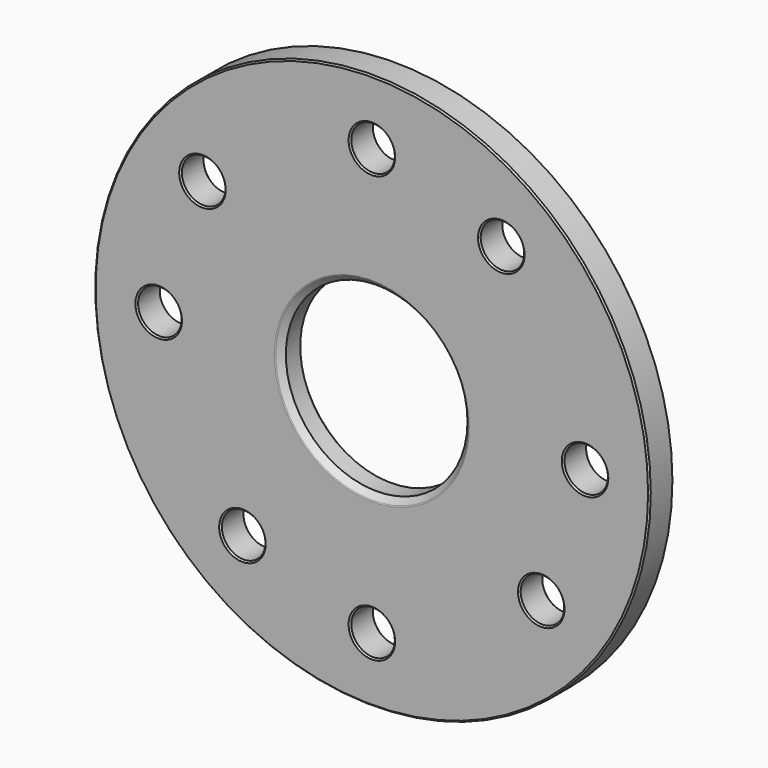
from build123d import *

# Parameters (mm, degrees)
F0_R     = 92.5
F0_R_2   = 7.25
F0_R_3   = 30.25
F1_DEPTH = 10
F2_SIZE2 = 2
F2_SIZE  = 2
F3_SIZE2 = 2
F3_SIZE  = 2


# Not quite as in the source:
# - a fillet or chamfer that OpenCascade refuses, or shapes differently, is made with other operations: its cross-section is extruded or revolved along the edge and cut away or added


with BuildPart() as f1:
    # F0 (on Front) → F1 (new body)
    with BuildSketch(Plane.XZ):
        Circle(F0_R)
        with BuildLine():
            ThreePointArc((-35.8509998507, -56.4207746479), (-35.9472026921, -57.5979263852), (-36.2332581163, -58.7438380282))
            ThreePointArc((-36.2332581163, -58.7438380282), (-50.2547970094, -55.2436229106), (-35.8509998507, -56.4207746479))
        make_face(mode=Mode.SUBTRACT)
        with BuildLine():
            ThreePointArc((-6.8677417345, -68.6769366197), (1.1771517373, -63.8462028413), (7.25, -71))
            ThreePointArc((7.25, -71), (-1.1771517373, -78.1537971587), (-6.8677417345, -68.6769366197))
        make_face(mode=Mode.SUBTRACT)
        with Locations((56.4207746479, -43.1009998507)):
            Circle(F0_R_2, mode=Mode.SUBTRACT)
        with Locations((-71, 0)):
            Circle(F0_R_2, mode=Mode.SUBTRACT)
        with Locations((-56.4207746479, 43.1009998507)):
            Circle(F0_R_2, mode=Mode.SUBTRACT)
        Circle(F0_R_3, mode=Mode.SUBTRACT)
        with Locations((71, 0)):
            Circle(F0_R_2, mode=Mode.SUBTRACT)
        with Locations((43.1009998507, 56.4207746479)):
            Circle(F0_R_2, mode=Mode.SUBTRACT)
        with Locations((0, 71)):
            Circle(F0_R_2, mode=Mode.SUBTRACT)
    extrude(amount=-F1_DEPTH)

    # F2
    f2_edges = [f1.edges().sort_by_distance(p)[0] for p in [
        (-30.25, 0, 0),
    ]]
    chamfer(f2_edges, length=F2_SIZE, length2=F2_SIZE2)

    # F3
    f3_edges = [f1.edges().sort_by_distance(p)[0] for p in [
        (-30.25, 10, 0),
    ]]
    chamfer(f3_edges, length=F3_SIZE, length2=F3_SIZE2)

    # F4: chamfer of 0.5 on 10 edges, made by hand

    # F4_s1 → F4_t2 (revolve, cut)
    with BuildSketch(Plane.XY):
        Polygon((32.1035533906, 9.8535533906), (32.4571067812, 10), (32.25, 10), align=None)
    revolve(axis=Axis((0, 10, 0), (0, -1, 0)), mode=Mode.SUBTRACT)

    # F4_s3 → F4_t4 (revolve, cut)
    with BuildSketch(Plane.XY):
        Polygon((92, 10), (92.5, 9.5), (92.5, 10), align=None)
    revolve(axis=Axis((0, 10, 0), (0, -1, 0)), mode=Mode.SUBTRACT)

    # F4_s5 → F4_t6 (revolve, cut)
    with BuildSketch(Plane.XY.offset(-56.4207746479)):
        Polygon((-35.3509998507, 10), (-35.8509998507, 9.5), (-35.8509998507, 10), align=None)
    revolve(axis=Axis((-43.1009998507, 10, -56.4207746479), (0, 1, 0)), mode=Mode.SUBTRACT)

    # F4_s7 → F4_t8 (revolve, cut)
    with BuildSketch(Plane(origin=(-21.5504999254, 0, -63.7103873239), x_dir=(0, 1, 0), z_dir=(-0.3204225352, 0, -0.947274722))):
        Polygon((10, 15), (9.5, 15.5), (10, 15.5), align=None)
    revolve(axis=Axis((0, 10, -71), (0, 1, 0)), mode=Mode.SUBTRACT)

    # F4_s9 → F4_t10 (revolve, cut)
    with BuildSketch(Plane.XY.offset(-43.1009998507)):
        Polygon((64.1707746479, 10), (63.6707746479, 9.5), (63.6707746479, 10), align=None)
    revolve(axis=Axis((56.4207746479, 10, -43.1009998507), (0, -1, 0)), mode=Mode.SUBTRACT)

    # F4_s11 → F4_t12 (revolve, cut)
    with BuildSketch(Plane.XY):
        Polygon((-63.25, 10), (-63.75, 9.5), (-63.75, 10), align=None)
    revolve(axis=Axis((-71, 10, 0), (0, -1, 0)), mode=Mode.SUBTRACT)

    # F4_s13 → F4_t14 (revolve, cut)
    with BuildSketch(Plane.XY.offset(43.1009998507)):
        Polygon((-48.6707746479, 10), (-49.1707746479, 9.5), (-49.1707746479, 10), align=None)
    revolve(axis=Axis((-56.4207746479, 10, 43.1009998507), (0, -1, 0)), mode=Mode.SUBTRACT)

    # F4_s15 → F4_t16 (revolve, cut)
    with BuildSketch(Plane.XY):
        Polygon((78.75, 10), (78.25, 9.5), (78.25, 10), align=None)
    revolve(axis=Axis((71, 10, 0), (0, -1, 0)), mode=Mode.SUBTRACT)

    # F4_s17 → F4_t18 (revolve, cut)
    with BuildSketch(Plane.XY.offset(56.4207746479)):
        Polygon((50.8509998507, 10), (50.3509998507, 9.5), (50.3509998507, 10), align=None)
    revolve(axis=Axis((43.1009998507, 10, 56.4207746479), (0, -1, 0)), mode=Mode.SUBTRACT)

    # F4_s19 → F4_t20 (revolve, cut)
    with BuildSketch(Plane.XY.offset(71)):
        Polygon((7.75, 10), (7.25, 9.5), (7.25, 10), align=None)
    revolve(axis=Axis((0, 10, 71), (0, -1, 0)), mode=Mode.SUBTRACT)

    # F5: chamfer of 0.5 on 10 edges, made by hand

    # F5_s1 → F5_t2 (revolve, cut)
    with BuildSketch(Plane.XY):
        Polygon((32.1035533906, 0.1464466094), (32.4571067812, 0), (32.25, 0), align=None)
    revolve(axis=Axis((0, 0, 0), (0, -1, 0)), mode=Mode.SUBTRACT)

    # F5_s3 → F5_t4 (revolve, cut)
    with BuildSketch(Plane.XY):
        Polygon((92, 0), (92.5, 0.5), (92.5, 0), align=None)
    revolve(axis=Axis((0, 0, 0), (0, -1, 0)), mode=Mode.SUBTRACT)

    # F5_s5 → F5_t6 (revolve, cut)
    with BuildSketch(Plane.XY.offset(-56.4207746479)):
        Polygon((-35.3509998507, 0), (-35.8509998507, 0.5), (-35.8509998507, 0), align=None)
    revolve(axis=Axis((-43.1009998507, 0, -56.4207746479), (0, -1, 0)), mode=Mode.SUBTRACT)

    # F5_s7 → F5_t8 (revolve, cut)
    with BuildSketch(Plane(origin=(-21.5504999254, 0, -63.7103873239), x_dir=(0, 1, 0), z_dir=(0.3204225352, 0, 0.947274722))):
        Polygon((0, -15), (0.5, -15.5), (0, -15.5), align=None)
    revolve(axis=Axis((0, 0, -71), (0, -1, 0)), mode=Mode.SUBTRACT)

    # F5_s9 → F5_t10 (revolve, cut)
    with BuildSketch(Plane.XY.offset(-43.1009998507)):
        Polygon((64.1707746479, 0), (63.6707746479, 0.5), (63.6707746479, 0), align=None)
    revolve(axis=Axis((56.4207746479, 0, -43.1009998507), (0, -1, 0)), mode=Mode.SUBTRACT)

    # F5_s11 → F5_t12 (revolve, cut)
    with BuildSketch(Plane.XY):
        Polygon((-63.25, 0), (-63.75, 0.5), (-63.75, 0), align=None)
    revolve(axis=Axis((-71, 0, 0), (0, -1, 0)), mode=Mode.SUBTRACT)

    # F5_s13 → F5_t14 (revolve, cut)
    with BuildSketch(Plane.XY.offset(43.1009998507)):
        Polygon((-48.6707746479, 0), (-49.1707746479, 0.5), (-49.1707746479, 0), align=None)
    revolve(axis=Axis((-56.4207746479, 0, 43.1009998507), (0, -1, 0)), mode=Mode.SUBTRACT)

    # F5_s15 → F5_t16 (revolve, cut)
    with BuildSketch(Plane.XY):
        Polygon((78.75, 0), (78.25, 0.5), (78.25, 0), align=None)
    revolve(axis=Axis((71, 0, 0), (0, -1, 0)), mode=Mode.SUBTRACT)

    # F5_s17 → F5_t18 (revolve, cut)
    with BuildSketch(Plane.XY.offset(56.4207746479)):
        Polygon((50.8509998507, 0), (50.3509998507, 0.5), (50.3509998507, 0), align=None)
    revolve(axis=Axis((43.1009998507, 0, 56.4207746479), (0, -1, 0)), mode=Mode.SUBTRACT)

    # F5_s19 → F5_t20 (revolve, cut)
    with BuildSketch(Plane.XY.offset(71)):
        Polygon((7.75, 0), (7.25, 0.5), (7.25, 0), align=None)
    revolve(axis=Axis((0, 0, 71), (0, -1, 0)), mode=Mode.SUBTRACT)


solid = f1.part
